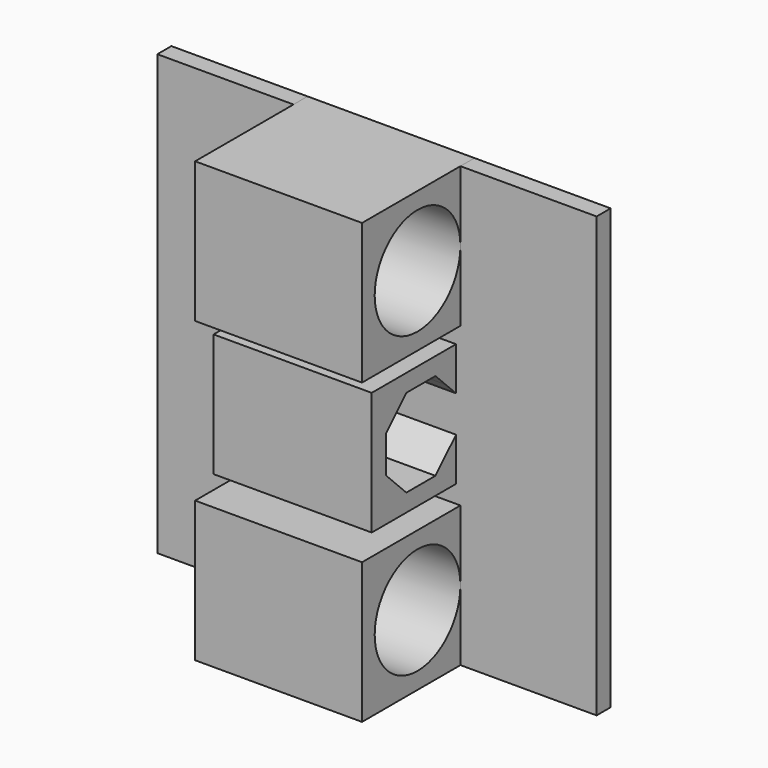
from build123d import *

# Parameters (mm, degrees)
F0_W     = 18
F0_H     = 14
F0_W_2   = 19
F0_H_2   = 16
F1_DEPTH = 2
F2_DEPTH = 14
F3_DEPTH = 16
F5_D     = 12.2
F7_D     = 12.2
F9_DEPTH = 25


# Not quite as in the source:
# - ends of sketch curves that miss each other by under 0.0002 mm in the source are joined


with BuildPart() as f1:
    # F0 (on Front) → F1 (new body)
    with BuildSketch(Plane.XZ):
        Polygon((9.5000003055, -25), (25, -25), (25, 25), (9.5000003055, 25), (9.5000003055, 8.9999977499), (-9.4999996945, 8.9999977499), (-9.4999996945, 24.9999977499), (-25, 25), (-25, -25), (-9.4999996945, -25), (-9.4999996945, -9), (9.5000003055, -9), align=None)
        Rectangle(F0_W, F0_H, mode=Mode.SUBTRACT)
        with Locations((3.055e-07, -17)):
            Rectangle(F0_W_2, F0_H_2)
        Polygon((9.5000003055, 8.9999977499), (9.5000003055, 24.9999977499), (-9.4999996945, 25), (-9.4999996945, 8.9999977499), align=None)
    extrude(amount=F1_DEPTH)

    # F0 (on Front) → F2 (join)
    with BuildSketch(Plane.XZ):
        Rectangle(F0_W, F0_H)
    extrude(amount=F2_DEPTH)

    # F0 (on Front) → F3 (join)
    with BuildSketch(Plane.XZ):
        with Locations((3.055e-07, -17)):
            Rectangle(F0_W_2, F0_H_2)
        Polygon((9.5000003055, 8.9999977499), (9.5000003055, 24.9999977499), (-9.4999996945, 25), (-9.4999996945, 8.9999977499), align=None)
    extrude(amount=F3_DEPTH)

    # F5 (through all)
    with Locations(Plane.YZ.offset(9.5000003055)):
        with Locations((-8.1, -17)):
            Hole(F5_D / 2)

    # F7 (through all)
    with Locations(Plane.YZ.offset(9.5000003055)):
        with Locations((-8.1, 16.9999977499)):
            Hole(F7_D / 2)

    # F8 (on face) → F9 (cut)
    with BuildSketch(Plane.YZ.offset(9)):
        with BuildLine():
            Line((-12.0000001043, -2.0710677001), (-10.5355339977, -3.5355338068))
            ThreePointArc((-10.5355339977, -3.5355338068), (-11.6193977653, -1.9134170539), (-12.0000001043, 1.212e-07))
            Line((-12.0000001043, 1.212e-07), (-12.0000001043, -2.0710677001))
        make_face()
        with BuildLine():
            ThreePointArc((-2.0000001043, 1.118e-07), (-2.3806024392, 1.9134172673), (-3.4644661888, 3.5355340081))
            ThreePointArc((-3.4644661888, 3.5355340081), (-5.0865829362, 4.6193977717), (-7.0000001043, 5.0000001118))
            ThreePointArc((-7.0000001043, 5.0000001118), (-8.9134172661, 4.6193977743), (-10.5355340102, 3.5355340177))
            ThreePointArc((-10.5355340102, 3.5355340177), (-11.6193977651, 1.9134172779), (-12.0000001043, 1.212e-07))
            ThreePointArc((-12.0000001043, 1.212e-07), (-11.6193977653, -1.9134170539), (-10.5355339977, -3.5355338068))
            ThreePointArc((-10.5355339977, -3.5355338068), (-8.9134172579, -4.6193975542), (-7.0000001043, -4.9999998882))
            ThreePointArc((-7.0000001043, -4.9999998882), (-5.0865829425, -4.6193975508), (-3.4644661984, -3.5355337942))
            ThreePointArc((-3.4644661984, -3.5355337942), (-2.3806024418, -1.9134170501), (-2.0000001043, 1.118e-07))
        make_face()
        with BuildLine():
            ThreePointArc((-12.0000001043, 1.212e-07), (-11.6193977651, 1.9134172779), (-10.5355340102, 3.5355340177))
            Line((-10.5355340102, 3.5355340177), (-12.0000001043, 2.0710679236))
            Line((-12.0000001043, 2.0710679236), (-12.0000001043, 1.212e-07))
        make_face()
        with BuildLine():
            ThreePointArc((-10.5355340102, 3.5355340177), (-8.9134172661, 4.6193977743), (-7.0000001043, 5.0000001118))
            Line((-7.0000001043, 5.0000001118), (-9.0710679162, 5.0000001118))
            Line((-9.0710679162, 5.0000001118), (-10.5355340102, 3.5355340177))
        make_face()
        with BuildLine():
            ThreePointArc((-7.0000001043, 5.0000001118), (-5.0865829362, 4.6193977717), (-3.4644661888, 3.5355340081))
            Line((-3.4644661888, 3.5355340081), (-4.9289322924, 5.0000001118))
            Line((-4.9289322924, 5.0000001118), (-7.0000001043, 5.0000001118))
        make_face()
        with BuildLine():
            Line((-3.4644661984, -3.5355337942), (-2.0000000522, -2.071067648))
            Line((-2.0000001043, -2.071067648), (-2.0000001043, 1.118e-07))
            ThreePointArc((-2.0000001043, 1.118e-07), (-2.3806024418, -1.9134170501), (-3.4644661984, -3.5355337942))
        make_face()
        with BuildLine():
            Line((-2.0000001043, 1.118e-07), (-2.0000001043, 2.0710678715))
            Line((-2.0000000522, 2.0710678715), (-3.4644661888, 3.5355340081))
            ThreePointArc((-3.4644661888, 3.5355340081), (-2.3806024392, 1.9134172673), (-2.0000001043, 1.118e-07))
        make_face()
        with BuildLine():
            Line((-4.9289322924, -4.9999998882), (-3.4644661984, -3.5355337942))
            ThreePointArc((-3.4644661984, -3.5355337942), (-5.0865829425, -4.6193975508), (-7.0000001043, -4.9999998882))
            Line((-7.0000001043, -4.9999998882), (-4.9289322924, -4.9999998882))
        make_face()
        with BuildLine():
            Line((-9.0710679162, -4.9999998882), (-7.0000001043, -4.9999998882))
            ThreePointArc((-7.0000001043, -4.9999998882), (-8.9134172579, -4.6193975542), (-10.5355339977, -3.5355338068))
            Line((-10.5355339977, -3.5355338068), (-9.0710679162, -4.9999998882))
        make_face()
    extrude(amount=-F9_DEPTH, mode=Mode.SUBTRACT)


solid = f1.part
